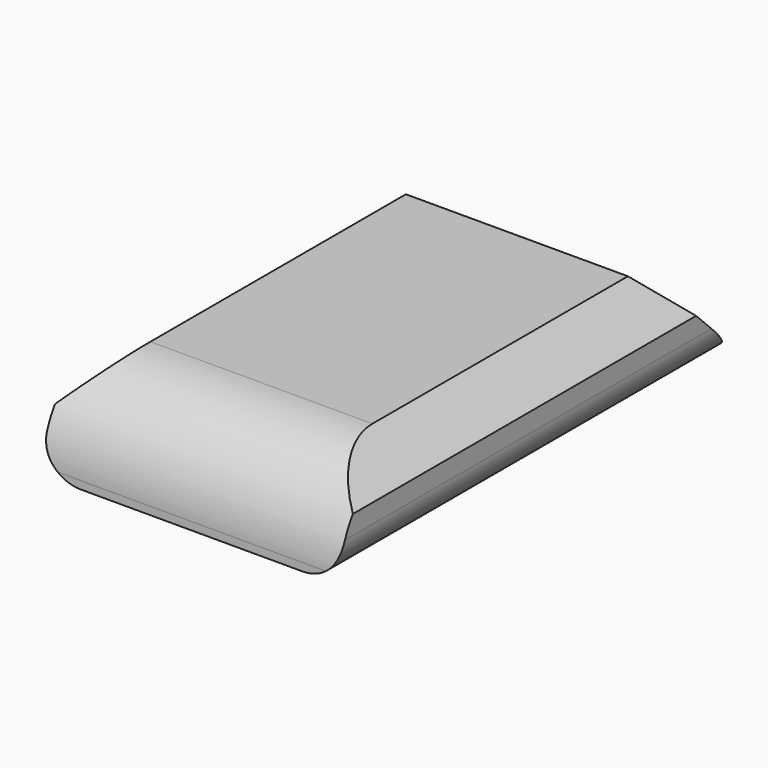
from build123d import *

# Parameters (mm, degrees)
F0_W        = 39.9140380323
F0_H        = 79.8528119922
F1_DEPTH    = 12.7
F2_T1_DEPTH = 170.555533821
F3_R        = 5.08
F4_SIZE     = 5.08
F5_R        = 11.650994652


# Not quite as in the source:
# - a fillet or chamfer that OpenCascade refuses, or shapes differently, is made with other operations: its cross-section is extruded or revolved along the edge and cut away or added


with BuildPart() as f1:
    # F0 (on Top) → F1 (new body)
    with BuildSketch(Plane.XY):
        with Locations((0, -6.916385144)):
            Rectangle(F0_W, F0_H)
    extrude(amount=F1_DEPTH)

    # F2: chamfer of 25.4 on 1 edges, made by hand

    # F2_s2 → F2_t1 (cut)
    with BuildSketch(Plane.YZ.offset(-85.2777669105)):
        Polygon((33.0100208521, -12.7), (7.6100208521, 12.7), (33.0100208521, 12.7), align=None)
    extrude(amount=F2_T1_DEPTH, mode=Mode.SUBTRACT)

    # F3
    f3_edges = [f1.edges().sort_by_distance(p)[0] for p in [
        (19.957019, -13.266385, 0),
        (-19.957019, -13.266385, 0),
    ]]
    fillet(f3_edges, radius=F3_R)

    # F4
    f4_edges = [f1.edges().sort_by_distance(p)[0] for p in [
        (-19.957019, -19.616385, 12.7),
        (19.957019, -19.616385, 12.7),
    ]]
    chamfer(f4_edges, length=F4_SIZE)

    # F5
    f5_edges = [f1.edges().sort_by_distance(p)[0] for p in [
        (0, -46.842791, 12.7),
    ]]
    fillet(f5_edges, radius=F5_R)


solid = f1.part
